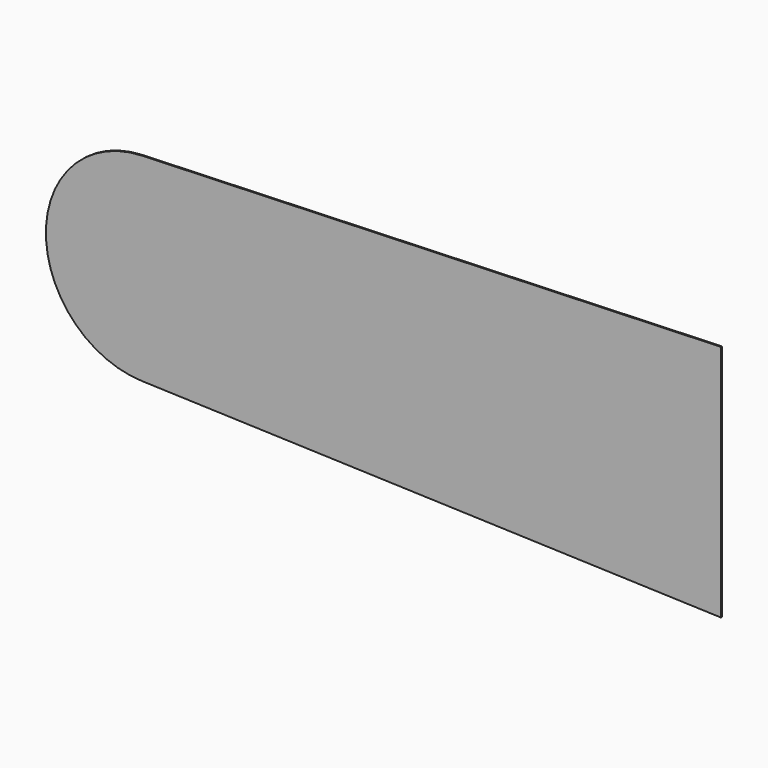
from build123d import *

# Parameters (mm, degrees)
F1_DEPTH = 0.75


# Not quite as in the source:
# - a feature names something its author has since deleted; it is built from what else it names


with BuildPart() as f1:
    # F0 (on Front) → F1 (new body, symmetric)
    with BuildSketch(Plane.XZ):
        with BuildLine():
            ThreePointArc((-729.2950732942, -124.9261875885), (-638.1434635786, -89.8940603204), (-600, 0))
            ThreePointArc((-600, 0), (-638.1434635786, 89.8940603204), (-729.2950732942, 124.9261875885))
            ThreePointArc((-729.2950732942, 124.9261875885), (-850, 0), (-729.2950732942, -124.9261875885))
        make_face()
        with BuildLine():
            Line((0, 0), (-600, 0))
            ThreePointArc((-600, 0), (-638.1434635786, -89.8940603204), (-729.2950732942, -124.9261875885))
            Line((-729.2950732942, -124.9261875885), (0, -150))
            Line((0, -150), (0, 0))
        make_face()
        with BuildLine():
            ThreePointArc((-729.2950732942, 124.9261875885), (-638.1434635786, 89.8940603204), (-600, 0))
            Line((-600, 0), (0, 0))
            Line((0, 0), (0, 150))
            Line((0, 150), (-729.2950732942, 124.9261875885))
        make_face()
    extrude(amount=F1_DEPTH, both=True)


solid = f1.part
